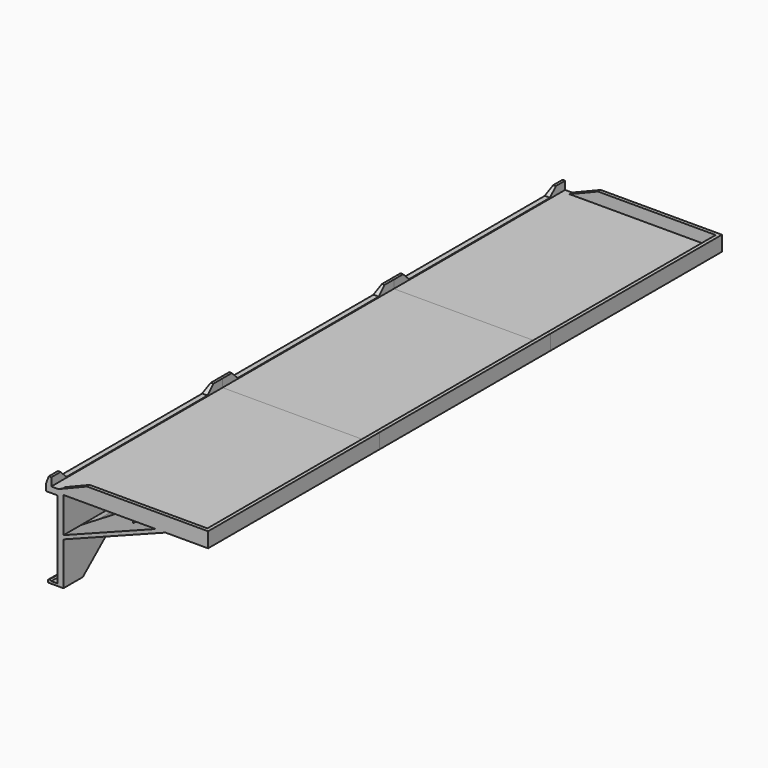
from build123d import *

# Parameters (mm, degrees)
F1_DEPTH  = 92.5
F3_DEPTH  = 4.501
F6_DEPTH  = 130.001
F8_DEPTH  = 10.001
F10_DEPTH = 3
F13_DEPTH = 3
F16_DEPTH = 6
F22_DEPTH = 10
F29_DEPTH = 3


with BuildPart() as f1:
    # F0 (on Front) → F1 (new body, symmetric)
    with BuildSketch(Plane.XZ):
        Polygon((4.7209845798, 31.831477772), (4.7209845798, -35.168522228), (-0.7790154202, -35.168522228), (-2.2790154202, -34.418522228), (-3.7790154202, -35.168522228), (-3.7790154202, -37.168522228), (9.7209845798, -37.168522228), (9.7209845798, 0), (97.8155508637, 33.831477772), (134.7209845798, 33.831477772), (134.7209845798, 36.831477772), (134.7209845798, 46.831477772), (131.7209845798, 46.831477772), (131.7209845798, 36.831477772), (9.7209845798, 36.831477772), (-0.7790154202, 36.831477772), (-0.7790154202, 43.831477772), (-3.0290154202, 43.831477772), (-5.2790154202, 37.831477772), (-5.2790154202, 31.831477772), align=None)
        Polygon((9.7209845798, 3.2136198107), (9.7209845798, 33.831477772), (89.4475320225, 33.831477772), align=None, mode=Mode.SUBTRACT)
    extrude(amount=F1_DEPTH, both=True)

    # F2 (on face) → F3 (cut, through all)
    with BuildSketch(Plane.YZ.offset(-0.7790154202)):
        Polygon((82.5, 43.831477772), (-82.5, 43.831477772), (-76.1718801937, 37.5033579657), (76.1718801937, 37.5033579657), align=None)
    extrude(amount=-F3_DEPTH, mode=Mode.SUBTRACT)

    # F5 (on face) → F6 (cut, through all)
    with BuildSketch(Plane(origin=(4.7209845798, 0, 0), x_dir=(0, -1, 0), z_dir=(-1, 0, 0))):
        Polygon((-271.3123908639, -49.6887229383), (-98.6876091361, -49.6887229383), (-185, 23.5453192145), align=None)
        Polygon((0, 23.5453192145), (-69.1991303871, -35.168522228), (69.1991303871, -35.168522228), align=None)
        Polygon((-69.1991303871, -35.168522228), (-86.3123908639, -49.6887229383), (86.3123908639, -49.6887229383), (69.1991303871, -35.168522228), align=None)
        Polygon((185, 23.5453192145), (98.6876091361, -49.6887229383), (271.3123908639, -49.6887229383), align=None)
    extrude(amount=-F6_DEPTH, mode=Mode.SUBTRACT)

    # F7 (on face) → F8 (cut, through all)
    with BuildSketch(Plane(origin=(4.7209845798, 0, 0), x_dir=(0, -1, 0), z_dir=(-1, 0, 0))):
        Polygon((67.8645954987, -34.0362006309), (-67.8645954987, -34.0362006309), (-69.1991303871, -35.168522228), (-71.9436615403, -37.4971926327), (71.9436615403, -37.4971926327), (69.1991303871, -35.168522228), align=None)
        Polygon((256.9436615403, -37.4971926327), (252.8645954987, -34.0362006309), (117.1354045013, -34.0362006309), (113.0563384597, -37.4971926327), align=None)
    extrude(amount=F8_DEPTH, mode=Mode.SUBTRACT)

    # F9 (on face) → F10 (cut)
    with BuildSketch(Plane(origin=(1.2494171556, 0, -3.253386186), x_dir=(0.9335267321, 0, 0.358507797), z_dir=(0.358507797, 0, -0.9335267321))):
        Polygon((9.0747989673, 27.75011095), (74.7506905709, 0), (9.0747989673, 74.6641680598), align=None)
        Polygon((9.0747989673, -74.6641680598), (74.7506905709, 0), (9.0747989673, -27.75011095), align=None)
        Polygon((9.0747989673, -27.75011095), (74.7506905709, 0), (9.0747989673, 27.75011095), align=None)
    extrude(amount=-F10_DEPTH, mode=Mode.SUBTRACT)


with BuildPart() as f11_1:
    # F11: instance of F1
    add(f1.part.mirror(Plane.XZ.offset(92.5)))

    # F12 (on face) → F13 (join)
    with BuildSketch(Plane.XZ.offset(277.5)):
        Polygon((24.1975653917, 46.831477772), (5.7930727489, 36.831477772), (131.7209845798, 36.831477772), (131.7209845798, 46.831477772), align=None)
    extrude(amount=-F13_DEPTH)


with BuildPart() as f14_1:
    # F14: instance of F11_1
    add(f11_1.part.mirror(Plane.XZ))


with BuildPart() as f1_1:
    add(f1.part)

    # F15 (on face) → F16 (cut)
    with BuildSketch(Plane(origin=(0, 0, -37.168522228), x_dir=(1, 0, 0), z_dir=(0, 0, -1))):
        Polygon((-3.7790154202, 67.8401216865), (4.6569141559, 69.272890687), (2.6162403041, 71.5562962167), (-3.7790154202, 71.5562962167), align=None)
        Polygon((-3.7790154202, 71.5562962167), (2.6162403041, 71.5562962167), (-3.7790154202, 78.7122473121), align=None)
        Polygon((-3.7790154202, -78.7122473121), (4.6569141559, -69.272890687), (-3.7790154202, -67.8401216865), align=None)
    extrude(amount=-F16_DEPTH, mode=Mode.SUBTRACT)


with BuildPart() as f19_1:
    # F19: instance of F1
    add(f1_1.part.mirror(Plane.XZ.offset(92.5)))


with BuildPart() as f20_1:
    # F20: instance of F19_1
    add(f19_1.part.mirror(Plane.XZ))


with BuildPart() as f1_2:
    add(f1_1.part)

    # F21 (on face) → F22 (cut)
    with BuildSketch(Plane(origin=(1.2494171556, 0, -3.253386186), x_dir=(0.9335267321, 0, 0.358507797), z_dir=(0.358507797, 0, -0.9335267321))):
        Polygon((44.5302129996, 57.0676339909), (61.6160072386, 37.6435107494), (61.6160072386, 77.5), align=None)
        Polygon((44.5302129996, -57.0676339909), (61.6160072386, -77.5), (61.6160072386, -37.6435107494), align=None)
    extrude(amount=-F22_DEPTH, mode=Mode.SUBTRACT)


with BuildPart() as f25_1:
    # F25: instance of F1
    add(f1_2.part.mirror(Plane.XZ.offset(92.5)))


with BuildPart() as f26_1:
    # F26: instance of F25_1
    add(f25_1.part.mirror(Plane.XZ))


with BuildPart() as f25_1_1:
    add(f25_1.part)

    # F28 (on face) → F29 (join)
    with BuildSketch(Plane.XZ.offset(277.5)):
        Polygon((30.0316457214, 46.831477772), (5.4077091627, 36.831477772), (131.7209845798, 36.831477772), (131.7209845798, 46.831477772), align=None)
    extrude(amount=-F29_DEPTH)


with BuildPart() as f30_1:
    # F30: instance of F25_1
    add(f25_1_1.part.mirror(Plane.XZ))


solid = Compound([f1_2.part, f25_1_1.part, f30_1.part])
